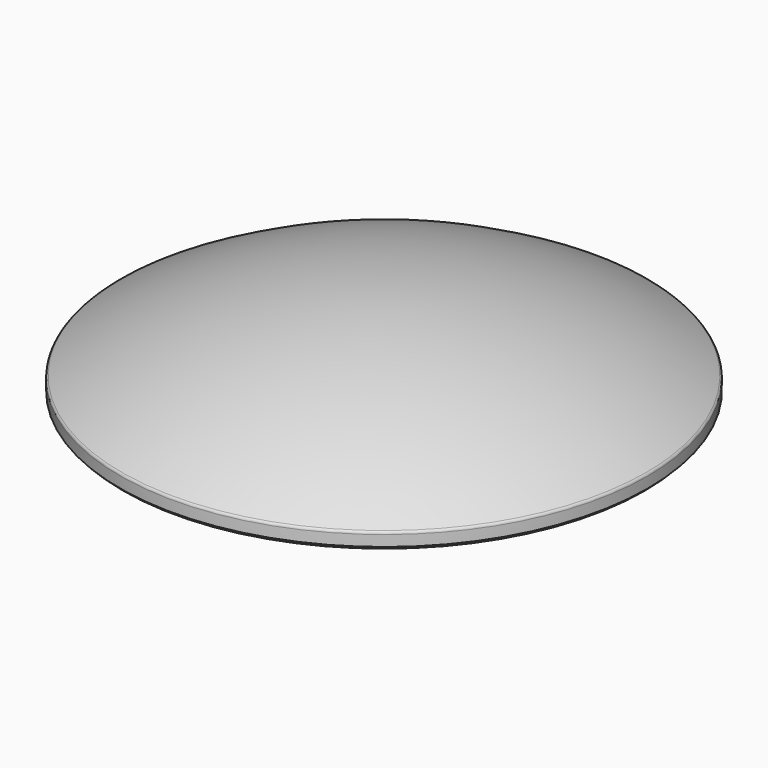
from build123d import *

# Parameters (mm, degrees)
F3_R = 0.1


# Not quite as in the source:
# - a fillet or chamfer that OpenCascade refuses, or shapes differently, is made with other operations: its cross-section is extruded or revolved along the edge and cut away or added


with BuildPart() as f1:
    # F0 (on Front) → F1 (revolve)
    with BuildSketch(Plane.XZ):
        with BuildLine():
            Line((5, 0), (8.3, 0))
            Line((8.3, 0), (8.3, 0.5))
            ThreePointArc((8.3, 0.5), (4.3063906, 2.2143660784), (0, 2.8))
            Line((0, 2.8), (0, 0.7))
            Line((0, 0.7), (4.4, 0.7))
            Line((4.4, 0.7), (5, 0))
        make_face()
    revolve(axis=Axis((0, 0, 0.2605222398), (0, 0, -1)))

    # F2: chamfer of 0.1 on 3 edges, made by hand

    # F2_s1 → F2_t2 (revolve)
    with BuildSketch(Plane.XZ):
        Polygon((4.3540065078, 0.7), (4.429932168, 0.6650791373), (4.4, 0.7), align=None)
    revolve(axis=Axis((0, 0, 0.7), (0, 0, -1)))

    # F2_s3 → F2_t4 (revolve, cut)
    with BuildSketch(Plane.XZ):
        Polygon((8.2, 0), (8.3, 0.1), (8.3, 0), align=None)
    revolve(axis=Axis((0, 0, 0), (0, 0, -1)), mode=Mode.SUBTRACT)

    # F2_s5 → F2_t6 (revolve, cut)
    with BuildSketch(Plane.XZ):
        Polygon((5.0459934922, 0), (4.970067832, 0.0349208627), (5, 0), align=None)
    revolve(axis=Axis((0, 0, 0), (0, 0, -1)), mode=Mode.SUBTRACT)

    # F3
    f3_edges = [f1.edges().sort_by_distance(p)[0] for p in [
        (-8.3, 0, 0.5),
    ]]
    fillet(f3_edges, radius=F3_R)


solid = f1.part
